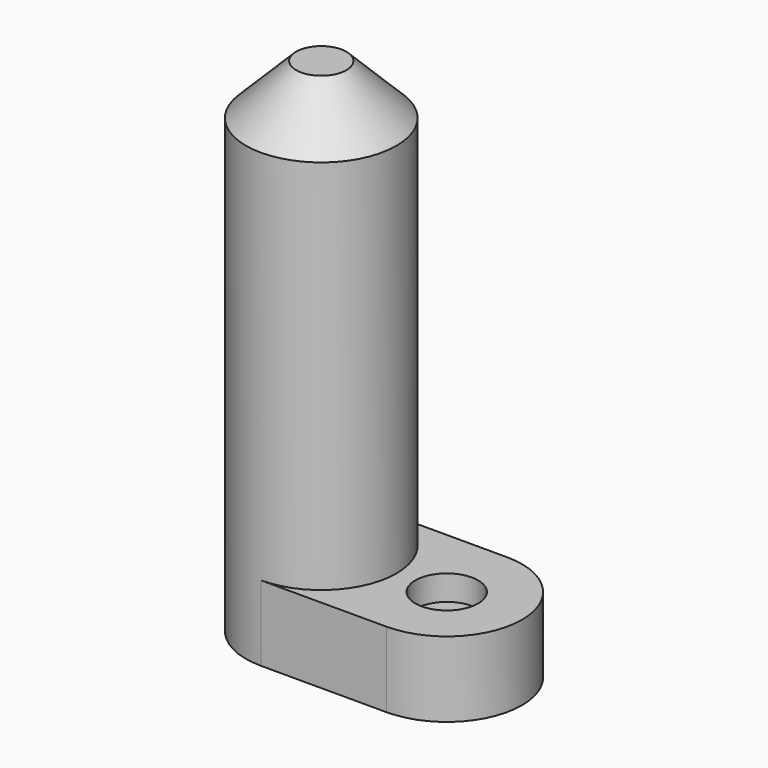
from build123d import *

# Parameters (mm, degrees)
F1_DEPTH = 50
F0_R     = 3.125
F2_DEPTH = 7.5
F0_R_2   = 1.625
F3_DEPTH = 5


# Not quite as in the source:
# - a fillet or chamfer that OpenCascade refuses, or shapes differently, is made with other operations: its cross-section is extruded or revolved along the edge and cut away or added


with BuildPart() as f1:
    # F0 (on Top) → F1 (new body)
    with BuildSketch(Plane.XY):
        with BuildLine():
            ThreePointArc((0, -7.5), (5.3033008589, -5.3033008589), (7.5, 0))
            ThreePointArc((7.5, 0), (5.3033008589, 5.3033008589), (0, 7.5))
            ThreePointArc((0, 7.5), (-7.5, 0), (0, -7.5))
        make_face()
    extrude(amount=F1_DEPTH)

    # F0 (on Top) → F2 (join)
    with BuildSketch(Plane.XY):
        with BuildLine():
            ThreePointArc((0, 7.5), (5.3033008589, 5.3033008589), (7.5, 0))
            ThreePointArc((7.5, 0), (5.3033008589, -5.3033008589), (0, -7.5))
            Line((0, -7.5), (12.5, -7.5))
            ThreePointArc((12.5, -7.5), (17.8033008589, -5.3033008589), (20, 0))
            ThreePointArc((20, 0), (17.8033008589, 5.3033008589), (12.5, 7.5))
            Line((12.5, 7.5), (0, 7.5))
        make_face()
        with Locations((12.5, 0)):
            Circle(F0_R, mode=Mode.SUBTRACT)
    extrude(amount=F2_DEPTH)

    # F0 (on Top) → F3 (join)
    with BuildSketch(Plane.XY):
        with Locations((12.5, 0)):
            Circle(F0_R)
        with Locations((12.5, 0)):
            Circle(F0_R_2, mode=Mode.SUBTRACT)
    extrude(amount=F3_DEPTH)

    # F4: chamfer of 5 on 1 edges, made by hand

    # F4_s1 → F4_t2 (revolve, cut)
    with BuildSketch(Plane.YZ):
        Polygon((-7.5, 45), (-2.5, 50), (-7.5, 50), align=None)
    revolve(axis=Axis((0, 0, 50), (0, 0, -1)), mode=Mode.SUBTRACT)


solid = f1.part
